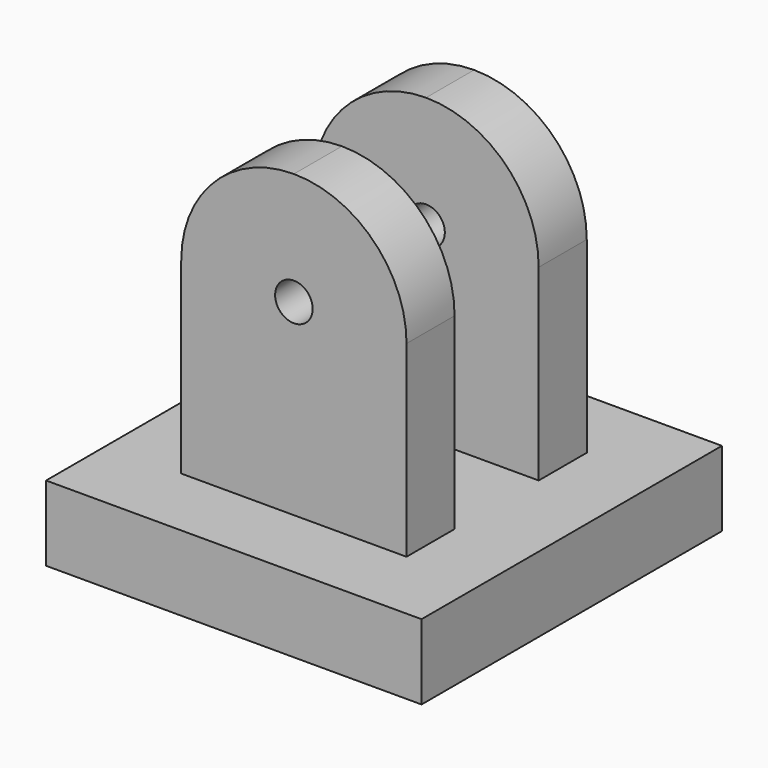
from build123d import *

# Parameters (mm, degrees)
F0_W     = 50
F0_H     = 50
F1_DEPTH = 10
F2_W     = 30
F2_H     = 8
F4_DEPTH = 40
F3_W     = 30
F3_H     = 8
F5_DEPTH = 40
F6_R     = 15
F7_R     = 15
F8_R     = 14.99999
F9_R     = 14.99999
F11_D    = 5


# Not quite as in the source:
# - a fillet or chamfer is up to 0.001 mm smaller than in the source, because OpenCascade refuses the exact size


with BuildPart() as f1:
    # F0 (on Top) → F1 (new body)
    with BuildSketch(Plane.XY):
        with Locations((2.0507174658, -2.8981622308)):
            Rectangle(F0_W, F0_H)
    extrude(amount=F1_DEPTH)

    # F2 (on face) → F4 (join)
    with BuildSketch(Plane.XY.offset(10)):
        with Locations((2.0507174658, 8.1018377692)):
            Rectangle(F2_W, F2_H)
    extrude(amount=F4_DEPTH)

    # F3 (on face) → F5 (join)
    with BuildSketch(Plane.XY.offset(10)):
        with Locations((2.0507174658, -13.8981622308)):
            Rectangle(F3_W, F3_H)
    extrude(amount=F5_DEPTH)

    # F6
    f6_edges = [f1.edges().sort_by_distance(p)[0] for p in [
        (17.050717, 8.101838, 50),
    ]]
    fillet(f6_edges, radius=F6_R)

    # F7
    f7_edges = [f1.edges().sort_by_distance(p)[0] for p in [
        (17.050717, -13.898162, 50),
    ]]
    fillet(f7_edges, radius=F7_R)

    # F8 (radius 15 in the source; OpenCascade refuses exactly that, so slightly less here)
    f8_edges = [f1.edges().sort_by_distance(p)[0] for p in [
        (-12.949283, 8.101838, 50),
    ]]
    fillet(f8_edges, radius=F8_R)

    # F9 (radius 15 in the source; OpenCascade refuses exactly that, so slightly less here)
    f9_edges = [f1.edges().sort_by_distance(p)[0] for p in [
        (-12.949283, -13.898162, 50),
    ]]
    fillet(f9_edges, radius=F9_R)

    # F11 (through all)
    with Locations(Plane(origin=(0, 12.1018377692, 0), x_dir=(-1, 0, 0), z_dir=(0, 1, 0))):
        with Locations((-2.0507174658, 35)):
            Hole(F11_D / 2)


solid = f1.part
